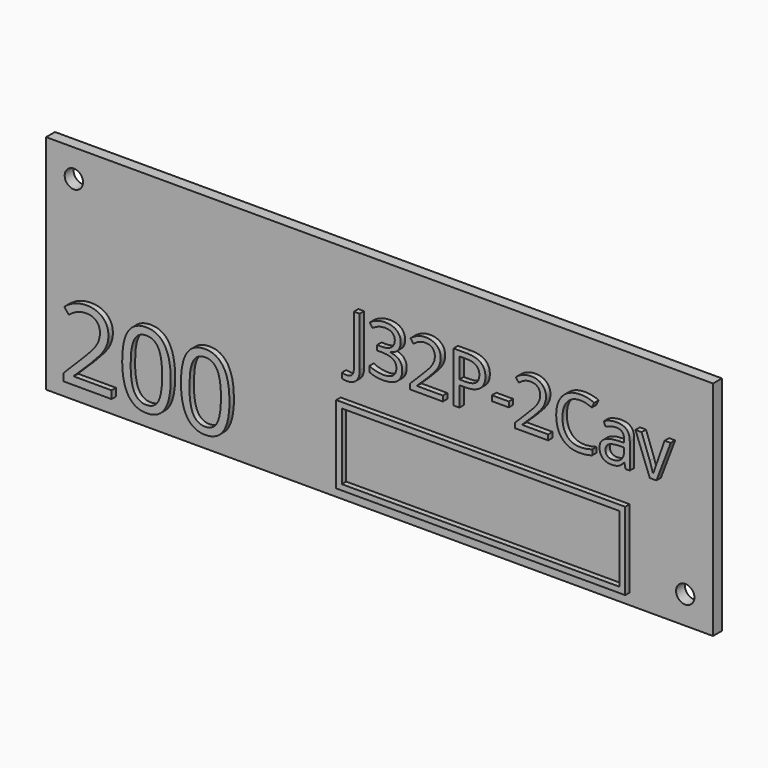
from build123d import *

# Parameters (mm, degrees)
F0_W         = 120
F0_H         = 40
F1_DEPTH     = 2
F3_D         = 3.3
F4_TEXT_SIZE = 12.6665787043
F5_DEPTH     = 1
F6_TEXT_SIZE = 18.4937691891
F7_DEPTH     = 1
F8_W         = 52
F8_H         = 14
F8_W_2       = 49.99999962
F8_H_2       = 11.99999962
F9_DEPTH     = 1


# Not quite as in the source:
# - Text() gives the source's letters only with a copy of the font that has no kerning and outlines rounded to 1/6400 em; it was checked with that copy


with BuildPart() as f1:
    # F0 (on Front) → F1 (new body)
    with BuildSketch(Plane.XZ):
        Rectangle(F0_W, F0_H)
    extrude(amount=F1_DEPTH)

    # F3 (through all)
    with Locations(Plane.XZ.offset(2)):
        with Locations((-55, 15), (55, -15)):
            Hole(F3_D / 2)

    # F4 (on face) → F5 (join)
    with BuildSketch(Plane.XZ.offset(2)):
        with Locations((-5, 2)):
            Text('J32P-2Cav', F4_TEXT_SIZE, font='Open Sans', text_align=(TextAlign.LEFT, TextAlign.BOTTOM))
    extrude(amount=F5_DEPTH)

    # F6 (on face) → F7 (join)
    with BuildSketch(Plane.XZ.offset(2)):
        with Locations((-57, -17)):
            Text('200', F6_TEXT_SIZE, font='Open Sans', text_align=(TextAlign.LEFT, TextAlign.BOTTOM))
    extrude(amount=F7_DEPTH)

    # F8 (on face) → F9 (join)
    with BuildSketch(Plane.XZ.offset(2)):
        with Locations((19, -11)):
            Rectangle(F8_W, F8_H)
        with Locations((19, -11)):
            Rectangle(F8_W_2, F8_H_2, mode=Mode.SUBTRACT)
    extrude(amount=F9_DEPTH)


solid = f1.part
